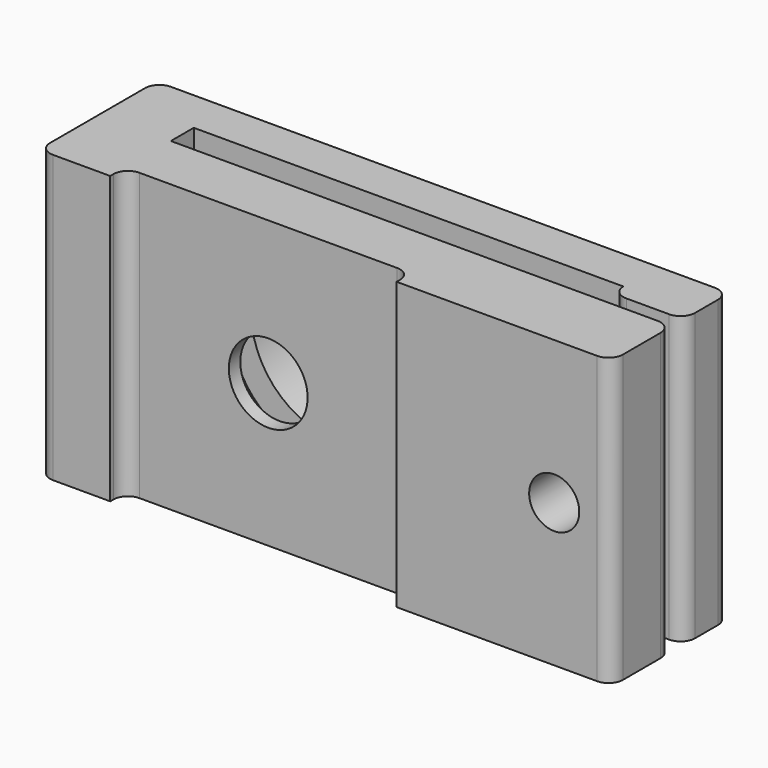
from build123d import *

# Parameters (mm, degrees)
F0_W     = 5
F0_H     = 2
F0_H_2   = 1.2903230384
F0_W_2   = 15
F0_H_3   = 1
F1_DEPTH = 20
F2_R     = 2.75
F2_R_2   = 1.75
F3_DEPTH = 25
F4_R     = 0.99999
F5_R     = 6
F5_R_2   = 2.75
F6_DEPTH = 5
F7_SIZE  = 3


# Not quite as in the source:
# - a fillet or chamfer is up to 0.001 mm smaller than in the source, because OpenCascade refuses the exact size


with BuildPart() as f1:
    # F0 (on Top) → F1 (new body)
    with BuildSketch(Plane.XY):
        Polygon((27.1122940337, 4), (-12.8877059663, 4), (-12.8877059663, 1), (-7.8877059663, 1), (22.1122940337, 1), (27.1122940337, 1), align=None)
        with Locations((-10.3877059663, 0)):
            Rectangle(F0_W, F0_H)
        Polygon((-7.8877059663, -1), (-12.8877059663, -1), (-12.8877059663, -5), (-7.8877059663, -5), (12.1122940337, -5), (27.1122940337, -5), (27.1122940337, -1), align=None)
        with Locations((-10.3877059663, -5.6451615192)):
            Rectangle(F0_W, F0_H_2)
        with Locations((19.6122940337, -5.6451615192)):
            Rectangle(F0_W_2, F0_H_2)
        with Locations((24.6122940337, 0.5)):
            Rectangle(F0_W, F0_H_3)
    extrude(amount=F1_DEPTH)

    # F2 (on face) → F3 (cut)
    with BuildSketch(Plane(origin=(0, 4, 0), x_dir=(-1, 0, 0), z_dir=(0, 1, 0))):
        with Locations((-2.1122940337, 10)):
            Circle(F2_R)
        with Locations((-23.1122940337, 10)):
            Circle(F2_R_2)
    extrude(amount=-F3_DEPTH, mode=Mode.SUBTRACT)

    # F4 (radius 1 in the source; OpenCascade refuses exactly that, so slightly less here)
    f4_edges = [f1.edges().sort_by_distance(p)[0] for p in [
        (-7.887706, -5, 10),
        (12.112294, -5, 10),
        (-12.887706, -6.290323, 10),
        (27.112294, -6.290323, 10),
        (27.112294, -1, 10),
        (27.112294, 0, 10),
        (27.112294, 4, 10),
        (-12.887706, 4, 10),
        (22.112294, 0, 15.71807),
        (22.112294, 0, 4.28193),
    ]]
    fillet(f4_edges, radius=F4_R)

    # F5 (on face) → F6 (cut)
    with BuildSketch(Plane(origin=(0, 4, 0), x_dir=(-1, 0, 0), z_dir=(0, 1, 0))):
        with Locations((-2.1122940337, 10)):
            Circle(F5_R)
        with Locations((-2.1122940337, 10)):
            Circle(F5_R_2, mode=Mode.SUBTRACT)
    extrude(amount=-F6_DEPTH, mode=Mode.SUBTRACT)

    # F7
    f7_edges = [f1.edges().sort_by_distance(p)[0] for p in [
        (4.862294, -1, 10),
    ]]
    chamfer(f7_edges, length=F7_SIZE)


solid = f1.part
